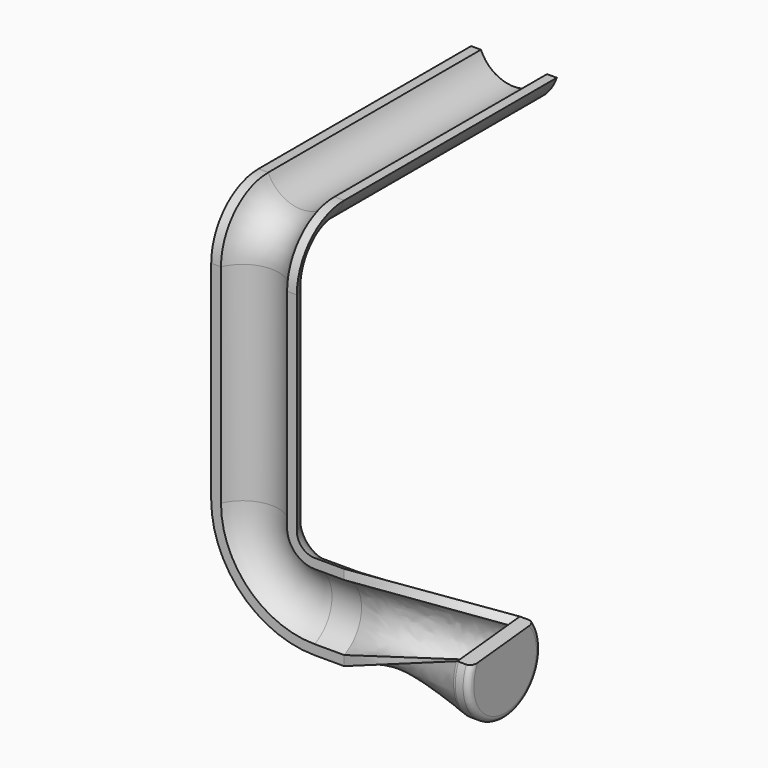
from build123d import *

# Parameters (mm, degrees)
F9_DEPTH = 5
F10_R    = 2


with BuildPart() as f2:
    # F2: sweep along a path in F1
    with BuildLine(Plane.YZ) as f2_path:
        Line((0, 0), (0, 45))
        ThreePointArc((0, 45), (5.8578643763, 59.1421356237), (20, 65))
        Line((20, 65), (110, 65))
    # F0 (on Top) → F2 (sweep)
    with BuildSketch(Plane.XY):
        with BuildLine():
            ThreePointArc((14, 0), (-0.5, 10.478936224), (-15, 0))
            Line((-15, 0), (-11.6882403352, 0))
            ThreePointArc((-11.6882403352, 0), (-0.5, 7.3789365762), (10.6882403352, 0))
            Line((10.6882403352, 0), (14, 0))
        make_face()
    sweep(path=f2_path.line)

    # F6: sweep along a path in F4
    with BuildLine(Plane.XZ) as f6_path:
        Line((0, 0), (0, -25.4587277886))
        ThreePointArc((0, -25.4587277886), (5.8578643763, -39.6008634124), (20, -45.4587277886))
        Line((20, -45.4587277886), (30, -45.4587277886))
    # F0 (on Top) → F6 (sweep)
    with BuildSketch(Plane.XY):
        with BuildLine():
            ThreePointArc((14, 0), (-0.5, 10.478936224), (-15, 0))
            Line((-15, 0), (-11.6882403352, 0))
            ThreePointArc((-11.6882403352, 0), (-0.5, 7.3789365762), (10.6882403352, 0))
            Line((10.6882403352, 0), (14, 0))
        make_face()
    sweep(path=f6_path.line)

    # F6_face (on face) → F7 section 0
    with BuildSketch(Plane(origin=(30, 5.8470332672, -45.9587277886), x_dir=(0, 1, 0), z_dir=(1, 0, 0))):
        with BuildLine():
            Line((-5.8470332672, -11.1882403352), (-5.8470332672, -14.5))
            ThreePointArc((-5.8470332672, -14.5), (4.6319029568, 0), (-5.8470332672, 14.5))
            Line((-5.8470332672, 14.5), (-5.8470332672, 11.1882403352))
            ThreePointArc((-5.8470332672, 11.1882403352), (1.5319033089, 0), (-5.8470332672, -11.1882403352))
        make_face()
    # F5 (on offset) → F7 section 1
    with BuildSketch(Plane.YZ.offset(79.5)):
        with BuildLine():
            Line((-10.8751536487, -37.9657093932), (-13.9526978979, -37.2235111379))
            ThreePointArc((-13.9526978979, -37.2235111379), (1.4814826902, -58.6311098034), (12.4912671201, -34.6460340717))
            Line((12.4912671201, -34.6460340717), (10.1624930815, -36.7332008739))
            ThreePointArc((10.1624930815, -36.7332008739), (0.7118567894, -55.5823045887), (-10.8751536487, -37.9657093932))
        make_face()
    loft()

    # F5 (on offset) + F8 (on face) → F9 (join)
    with BuildSketch(Plane.YZ.offset(79.5)):
        with BuildLine():
            Line((-10.8751536487, -37.9657093932), (-13.9526978979, -37.2235111379))
            ThreePointArc((-13.9526978979, -37.2235111379), (1.4814826902, -58.6311098034), (12.4912671201, -34.6460340717))
            Line((12.4912671201, -34.6460340717), (10.1624930815, -36.7332008739))
            ThreePointArc((10.1624930815, -36.7332008739), (0.7118567894, -55.5823045887), (-10.8751536487, -37.9657093932))
        make_face()
    with BuildSketch(Plane.YZ.offset(79.5)):
        with BuildLine():
            Line((12.4912671201, -34.6460340717), (10.1624930815, -36.7332008739))
            ThreePointArc((10.1624930815, -36.7332008739), (0.7118567894, -55.5823045887), (-10.8751536487, -37.9657093932))
            Line((-10.8751536487, -37.9657093932), (-13.9526978979, -37.2235111379))
            ThreePointArc((-13.9526978979, -37.2235111379), (1.4814826902, -58.6311098034), (12.4912671201, -34.6460340717))
        make_face()
        with BuildLine():
            ThreePointArc((-10.8751536487, -37.9657093932), (0.7118567894, -55.5823045887), (10.1624930815, -36.7332008739))
            Line((10.1624930815, -36.7332008739), (12.4912671201, -34.6460340717))
            Line((12.4912671201, -34.6460340717), (-13.9526978979, -37.2235111379))
            Line((-13.9526978979, -37.2235111379), (-10.8751536487, -37.9657093932))
        make_face()
    extrude(amount=F9_DEPTH)

    # F10
    f10_edges = [f2.edges().sort_by_distance(p)[0] for p in [
        (84.5, 1.481483, -58.63111),
        (79.5, 1.481483, -58.63111),
    ]]
    fillet(f10_edges, radius=F10_R)


solid = f2.part
